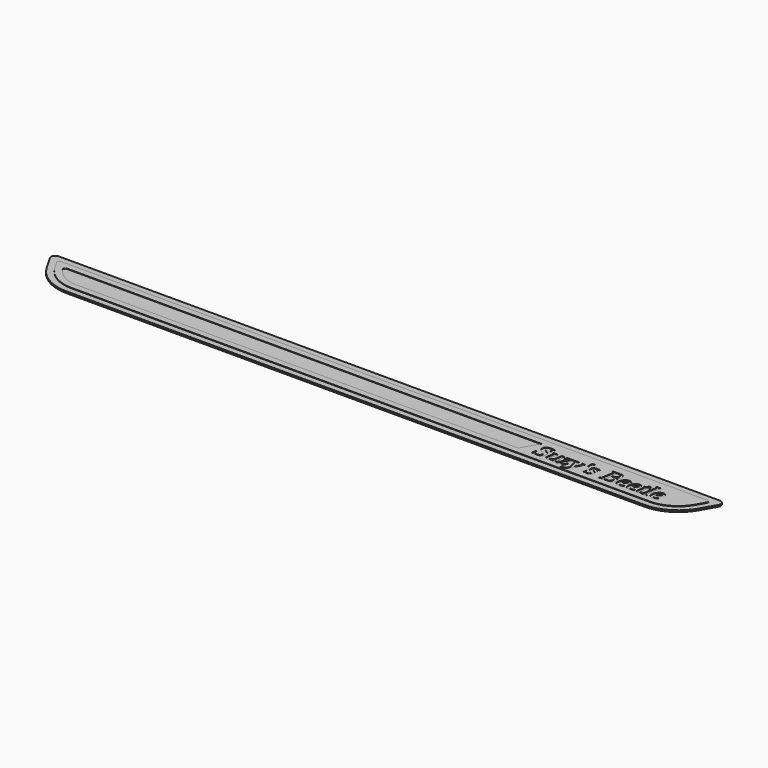
from build123d import *

# Parameters (mm, degrees)
F1_DEPTH     = 2
F3_DEPTH     = 0.5
F4_TEXT_SIZE = 27.7777777778
F5_DEPTH     = 0.5


# Not quite as in the source:
# - Text() gives the source's letters only with a copy of the font that has no kerning and outlines rounded to 1/6400 em; it was checked with that copy


with BuildPart() as f1:
    # F0 (on Top) → F1 (new body)
    with BuildSketch(Plane.XY):
        with BuildLine():
            Line((-340.9252271189, -25), (340.9252271189, -25))
            ThreePointArc((340.9252271189, -25), (365.9252271189, -18.3012701892), (384.2264973081, 0))
            Line((384.2264973081, 0), (394.3301270189, 17.5))
            ThreePointArc((394.3301270189, 17.5), (394.3301270189, 22.5), (390, 25))
            Line((390, 25), (-390, 25))
            ThreePointArc((-390, 25), (-394.3301270189, 22.5), (-394.3301270189, 17.5))
            Line((-394.3301270189, 17.5), (-384.2264973081, 0))
            ThreePointArc((-384.2264973081, 0), (-365.9252271189, -18.3012701892), (-340.9252271189, -25))
        make_face()
    extrude(amount=F1_DEPTH)


with BuildPart() as f3:
    # F2 (on face) → F3 (new body)
    with BuildSketch(Plane.XY.offset(2)):
        with BuildLine():
            ThreePointArc((340.9252271189, -17.5), (362.1752271189, -11.8060796608), (377.7313067797, 3.75))
            Line((377.7313067797, 3.75), (383.5048094716, 13.75))
            ThreePointArc((383.5048094716, 13.75), (383.5048094716, 16.25), (381.3397459622, 17.5))
            Line((381.3397459622, 17.5), (-381.3397459622, 17.5))
            ThreePointArc((-381.3397459622, 17.5), (-383.5048094716, 16.25), (-383.5048094716, 13.75))
            Line((-383.5048094716, 13.75), (-377.7313067797, 3.75))
            ThreePointArc((-377.7313067797, 3.75), (-362.1752271189, -11.8060796608), (-340.9252271189, -17.5))
            Line((-340.9252271189, -17.5), (340.9252271189, -17.5))
        make_face()
        with BuildLine():
            Line((-368.3113549941, 10), (191.5470053838, 10))
            Line((191.5470053838, 10), (180, -10))
            Line((180, -10), (-340.9252271189, -10))
            ThreePointArc((-340.9252271189, -10), (-357.7386832684, -5.6970306757), (-370.4179802153, 6.1538461538))
            ThreePointArc((-370.4179802153, 6.1538461538), (-370.5040000424, 8.7009611535), (-368.3113549941, 10))
        make_face(mode=Mode.SUBTRACT)
    extrude(amount=F3_DEPTH)

    # F4 (on face) → F5 (cut)
    with BuildSketch(Plane.XY.offset(2.5)):
        with Locations((195, -10)):
            Text("Suzy's Beetle", F4_TEXT_SIZE, font='Tinos', font_style=FontStyle.BOLDITALIC, text_align=(TextAlign.LEFT, TextAlign.BOTTOM))
    extrude(amount=-F5_DEPTH, mode=Mode.SUBTRACT)


solid = Compound([f1.part, f3.part])
